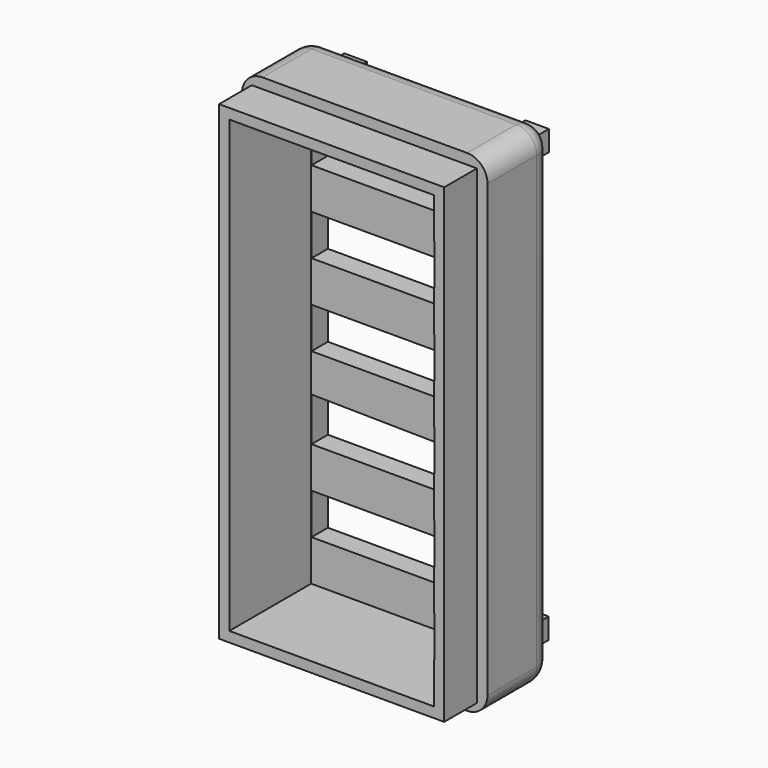
from build123d import *

# Parameters (mm, degrees)
F0_W      = 55
F0_H      = 115
F0_W_2    = 50
F0_H_2    = 110
F1_DEPTH  = 20
F3_W      = 55
F3_H      = 115
F5_DEPTH  = 10
F6_W      = 50
F6_H      = 110
F7_DEPTH  = 215.8
F8_W      = 60
F8_H      = 120
F9_DEPTH  = 5
F10_W     = 50
F10_H     = 10
F12_DEPTH = 30.001
F13_R     = 4.99999
F14_W     = 5.7372912765
F14_H     = 5
F14_W_2   = 5.2530970424
F14_H_2   = 5.0719603896
F15_DEPTH = 5
F16_W     = 5.5731512606
F16_H     = 5
F16_H_2   = 5.1789134741
F17_DEPTH = 5


# Not quite as in the source:
# - a fillet or chamfer is up to 0.001 mm smaller than in the source, because OpenCascade refuses the exact size


with BuildPart() as f1:
    # F0 (on Front) → F1 (new body)
    with BuildSketch(Plane.XZ):
        Polygon((-31.2259571254, 74.3091152272), (-33.7259571254, 74.3091152272), (-33.7259571254, -45.6908847728), (26.2740428746, -45.6908847728), (26.2740428746, 74.3091152272), align=None)
        with Locations((-3.7259571254, 14.3091152272)):
            Rectangle(F0_W, F0_H, mode=Mode.SUBTRACT)
        with Locations((-3.7259571254, 14.3091152272)):
            Rectangle(F0_W, F0_H)
        with Locations((-3.7259571254, 14.3091152272)):
            Rectangle(F0_W_2, F0_H_2, mode=Mode.SUBTRACT)
    extrude(amount=F1_DEPTH)

    # F3 (on offset) + F4 (on offset) → F5 (join)
    with BuildSketch(Plane.XZ.offset(20)):
        with Locations((-3.8123092055, 14.2757248878)):
            Rectangle(F3_W, F3_H)
    with BuildSketch(Plane.XZ.offset(20)):
        Polygon((-28.6821052432, -40.8934615552), (21.3168207556, -40.8934615552), (20.2441066504, 69.0581277013), (-28.6821052432, 69.0581277013), align=None)
    extrude(amount=F5_DEPTH)

    # F6 (on face) → F7 (cut)
    with BuildSketch(Plane.XZ.offset(30)):
        with Locations((-3.8123092055, 14.2757248878)):
            Rectangle(F6_W, F6_H)
    extrude(amount=-F7_DEPTH, mode=Mode.SUBTRACT)

    # F8 (on face) → F9 (join)
    with BuildSketch(Plane(origin=(0, 0, 0), x_dir=(-1, 0, 0), z_dir=(0, 1, 0))):
        with Locations((3.7259571254, 14.3091152272)):
            Rectangle(F8_W, F8_H)
    extrude(amount=-F9_DEPTH)

    # F10 (on face) → F12 (cut, through all)
    with BuildSketch(Plane(origin=(0, 0, 0), x_dir=(-1, 0, 0), z_dir=(0, 1, 0))):
        with Locations((3.7259571254, 54.3091152272)):
            Rectangle(F10_W, F10_H)
        with Locations((3.7259571254, 34.3091152272)):
            Rectangle(F10_W, F10_H)
        with Locations((3.7259571254, 14.3091152272)):
            Rectangle(F10_W, F10_H)
        Polygon((-21.2740428746, -0.6908847728), (-21.2740428746, -10.6908847728), (28.7259571254, -10.6908847728), (28.7259571254, 0), align=None)
        with Locations((3.7259571254, -25.6908847728)):
            Rectangle(F10_W, F10_H)
    extrude(amount=-F12_DEPTH, mode=Mode.SUBTRACT)

    # F13 (radius 5 in the source; OpenCascade refuses exactly that, so slightly less here)
    f13_edges = [f1.edges().sort_by_distance(p)[0] for p in [
        (-3.725957, 0, -45.690885),
        (-33.725957, 0, 14.309115),
        (26.274043, 0, 14.309115),
        (-3.725957, 0, 74.309115),
        (26.274043, -10, -45.690885),
        (26.274043, -10, 74.309115),
        (-33.725957, -10, -45.690885),
        (-33.725957, -10, 74.309115),
    ]]
    fillet(f13_edges, radius=F13_R)

    # F14 (on face) → F15 (join)
    with BuildSketch(Plane(origin=(0, 0, 0), x_dir=(-1, 0, 0), z_dir=(0, 1, 0))):
        with Locations((-18.4053972363, 66.8091152272)):
            Rectangle(F14_W, F14_H)
        with Locations((-18.5921611264, -38.1038859487)):
            Rectangle(F14_W_2, F14_H_2)
    extrude(amount=F15_DEPTH)

    # F16 (on face) → F17 (join)
    with BuildSketch(Plane(origin=(0, 0, 0), x_dir=(-1, 0, 0), z_dir=(0, 1, 0))):
        with Locations((25.9393814951, 66.8091152272)):
            Rectangle(F16_W, F16_H)
        with Locations((25.9393814951, -38.0802713335)):
            Rectangle(F16_W, F16_H_2)
    extrude(amount=F17_DEPTH)


solid = f1.part
